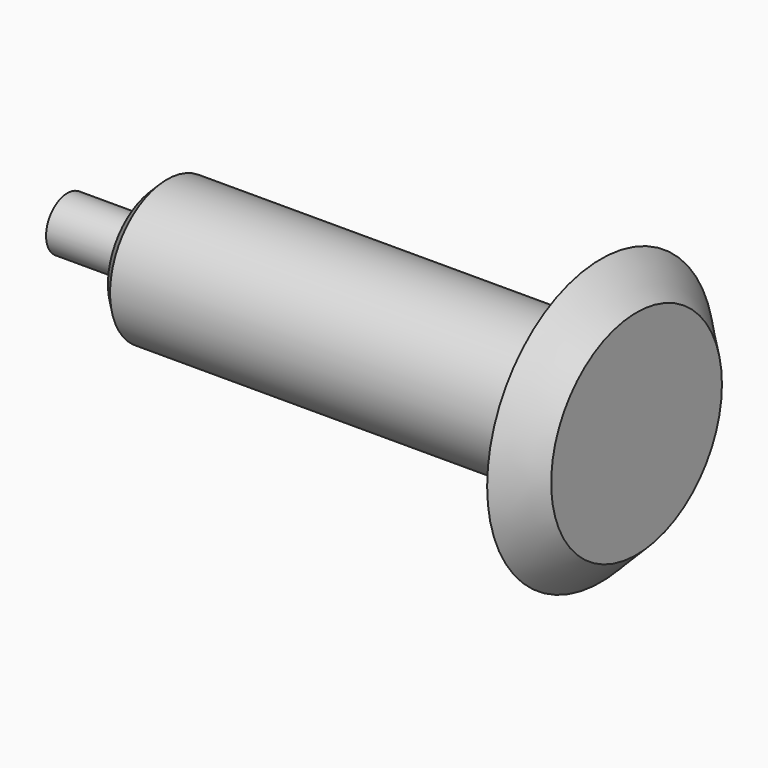
from build123d import *

# Parameters (mm, degrees)
F0_R        = 40
F0_R_2      = 25
F1_DEPTH    = 10
F0_R_3      = 20
F2_DEPTH    = 20
F0_R_4      = 7.5
F3_DEPTH    = 135
F4_DEPTH    = 160
F5_S8_R     = 20
F5_T9_DEPTH = 37
F6_SIZE2    = 3
F6_SIZE     = 3


# Not quite as in the source:
# - a fillet or chamfer that OpenCascade refuses, or shapes differently, is made with other operations: its cross-section is extruded or revolved along the edge and cut away or added


with BuildPart() as f1:
    # F0 (on Right) → F1 (new body)
    with BuildSketch(Plane.YZ):
        Circle(F0_R)
        Circle(F0_R_2, mode=Mode.SUBTRACT)
    extrude(amount=-F1_DEPTH)

    # F0 (on Right) → F2 (join)
    with BuildSketch(Plane.YZ):
        Circle(F0_R_2)
        Circle(F0_R_3, mode=Mode.SUBTRACT)
    extrude(amount=-F2_DEPTH)

    # F0 (on Right) → F3 (join)
    with BuildSketch(Plane.YZ):
        Circle(F0_R_3)
        Circle(F0_R_4, mode=Mode.SUBTRACT)
    extrude(amount=-F3_DEPTH)

    # F0 (on Right) → F4 (join)
    with BuildSketch(Plane.YZ):
        Circle(F0_R_4)
    extrude(amount=-F4_DEPTH)

    # F5: chamfer of 10 on 2 edges, made by hand

    # F5_s1 → F5_t2 (revolve, cut)
    with BuildSketch(Plane.XY):
        Polygon((-10, 40), (0, 30), (0, 40), align=None)
    revolve(axis=Axis((0, 0, 0), (1, 0, 0)), mode=Mode.SUBTRACT)


with BuildPart() as f5_tool4:
    # F5_s5 → F5_t6 (revolve)
    with BuildSketch(Plane.XY):
        Polygon((-10, 25), (-20, 15), (-20, 25), align=None)
    revolve(axis=Axis((-20, 0, 0), (1, 0, 0)))

    split(bisect_by=Plane.YZ.offset(-10), keep=Keep.BOTTOM)

    # F5_s8 → F5_t9 (cut, symmetric)
    with BuildSketch(Plane.YZ.offset(-15)):
        Circle(F5_S8_R)
    extrude(amount=F5_T9_DEPTH, both=True, mode=Mode.SUBTRACT)


with BuildPart() as f1_1:
    add(f1.part)

    # F5_t3: cut F5_tool4
    add(f5_tool4.part, mode=Mode.SUBTRACT)

    # F6
    f6_edges = [f1_1.edges().sort_by_distance(p)[0] for p in [
        (-135, -20, 0),
    ]]
    chamfer(f6_edges, length=F6_SIZE, length2=F6_SIZE2)


solid = f1_1.part
